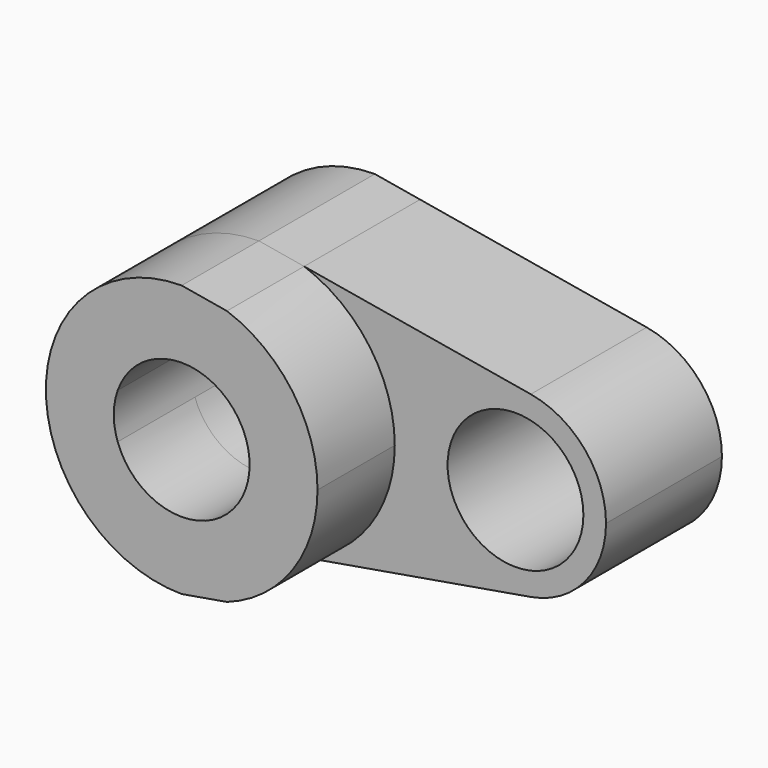
from build123d import *
from build123d import SkipClean  # not in build123d's __all__

# Parameters (mm, degrees)
F0_R     = 14.2875
F1_DEPTH = 30.48
F2_DEPTH = 50.8


with BuildPart() as f1:
    # F0 (on Front) → F1 (new body)
    with BuildSketch(Plane.XZ):
        with BuildLine():
            Line((9.5121844836, 26.9452959039), (0, 28.575))
            ThreePointArc((0, 28.575), (-28.575, 0), (0, -28.575))
            Line((0, -28.575), (9.5121844836, -26.9452959039))
            ThreePointArc((9.5121844836, -26.9452959039), (23.3274655355, -16.5033322905), (28.575, 0))
            ThreePointArc((28.575, 0), (23.3274655355, 16.5033322905), (9.5121844836, 26.9452959039))
        make_face()
        with BuildLine():
            ThreePointArc((-13.4703841816, 4.7625), (0, 14.2875), (13.4703841816, 4.7625))
            Line((13.4703841816, 4.7625), (19.05, 4.7625))
            Line((19.05, 4.7625), (19.05, -4.7625))
            Line((19.05, -4.7625), (13.4703841816, -4.7625))
            ThreePointArc((13.4703841816, -4.7625), (0, -14.2875), (-13.4703841816, -4.7625))
            Line((-13.4703841816, -4.7625), (-19.05, -4.7625))
            Line((-19.05, -4.7625), (-19.05, 4.7625))
            Line((-19.05, 4.7625), (-13.4703841816, 4.7625))
        make_face(mode=Mode.SUBTRACT)
        with BuildLine():
            Line((57.1919272622, 18.7764181619), (9.5121844836, 26.9452959039))
            ThreePointArc((9.5121844836, 26.9452959039), (23.3274655355, 16.5033322905), (28.575, 0))
            ThreePointArc((28.575, 0), (23.3274655355, -16.5033322905), (9.5121844836, -26.9452959039))
            Line((9.5121844836, -26.9452959039), (57.1919272622, -18.7764181619))
            ThreePointArc((57.1919272622, -18.7764181619), (34.925, 0), (57.1919272622, 18.7764181619))
        make_face()
        with BuildLine():
            ThreePointArc((73.025, 0), (68.5383952831, 12.2804730295), (57.1919272622, 18.7764181619))
            ThreePointArc((57.1919272622, 18.7764181619), (34.925, 0), (57.1919272622, -18.7764181619))
            ThreePointArc((57.1919272622, -18.7764181619), (68.5383952831, -12.2804730295), (73.025, 0))
        make_face()
        with Locations((53.975, 0)):
            Circle(F0_R, mode=Mode.SUBTRACT)
    extrude(amount=F1_DEPTH)

    # F0 (on Front) → F2 (join)
    with BuildSketch(Plane.XZ):
        with BuildLine():
            Line((9.5121844836, 26.9452959039), (0, 28.575))
            ThreePointArc((0, 28.575), (-28.575, 0), (0, -28.575))
            Line((0, -28.575), (9.5121844836, -26.9452959039))
            ThreePointArc((9.5121844836, -26.9452959039), (23.3274655355, -16.5033322905), (28.575, 0))
            ThreePointArc((28.575, 0), (23.3274655355, 16.5033322905), (9.5121844836, 26.9452959039))
        make_face()
        with BuildLine():
            ThreePointArc((-13.4703841816, 4.7625), (0, 14.2875), (13.4703841816, 4.7625))
            Line((13.4703841816, 4.7625), (19.05, 4.7625))
            Line((19.05, 4.7625), (19.05, -4.7625))
            Line((19.05, -4.7625), (13.4703841816, -4.7625))
            ThreePointArc((13.4703841816, -4.7625), (0, -14.2875), (-13.4703841816, -4.7625))
            Line((-13.4703841816, -4.7625), (-19.05, -4.7625))
            Line((-19.05, -4.7625), (-19.05, 4.7625))
            Line((-19.05, 4.7625), (-13.4703841816, 4.7625))
        make_face(mode=Mode.SUBTRACT)
        with BuildLine():
            ThreePointArc((-13.4703841816, -4.7625), (-14.2875, 0), (-13.4703841816, 4.7625))
            Line((-13.4703841816, 4.7625), (-19.05, 4.7625))
            Line((-19.05, 4.7625), (-19.05, -4.7625))
            Line((-19.05, -4.7625), (-13.4703841816, -4.7625))
        make_face()
        with BuildLine():
            ThreePointArc((13.4703841816, 4.7625), (14.081739421, 2.416044521), (14.2875, 0))
            ThreePointArc((14.2875, 0), (14.081739421, -2.416044521), (13.4703841816, -4.7625))
            Line((13.4703841816, -4.7625), (19.05, -4.7625))
            Line((19.05, -4.7625), (19.05, 4.7625))
            Line((19.05, 4.7625), (13.4703841816, 4.7625))
        make_face()
    with SkipClean():  # cleaning this boolean's faces spoils the solid; the shape is the same uncleaned
        extrude(amount=F2_DEPTH)


solid = f1.part
